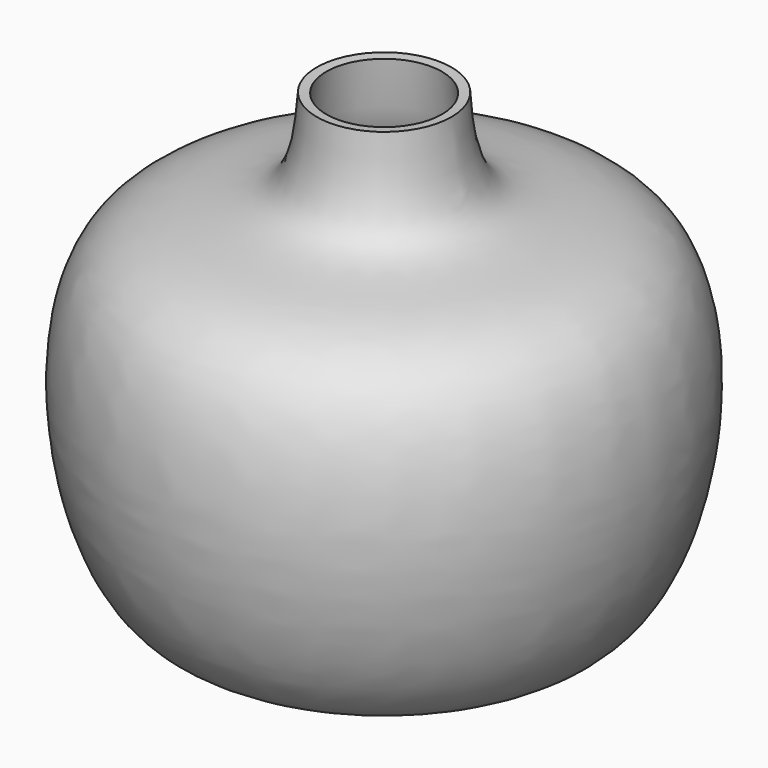
from build123d import *


# Not quite as in the source:
# - ends of sketch curves that miss each other by under 0.0002 mm in the source are joined
# - the dataset's text gives a spline's control points without its knots; the knots are read off the source's solid


with BuildPart() as f1:
    # F0 (on Front) → F1 (revolve)
    with BuildSketch(Plane.XZ):
        with BuildLine():
            add(Edge.make_bspline(
                [(0, 0), (12.2604930092, 0), (37.1680432505, -14.4897537862), (45.8159764504, 54.0703124701), (10.8709015607, 48.0211229848), (9.6057950827, 61.8857288852), (9.1015450487, 68.0656330135)],
                knots=[0, 0, 0, 0, 0.2642831779, 0.5818122538, 0.8089805027, 1, 1, 1, 1], degree=3))
            Line((0, 0), (0, -1.5000011719))
            add(Edge.make_bspline(
                [(0, -1.5000011719), (2.7725135208, -1.5000011719), (6.9145647776, -2.0308322394), (12.2903121109, -3.0792987233), (16.2230322301, -3.8437402004), (20.0419075684, -4.3880328646), (23.7428872911, -4.4983960181), (26.7225260222, -4.0210829824), (29.0016471213, -3.1616629238), (30.634715187, -2.2528712489), (32.1737960375, -1.0569174337), (33.5849093089, 0.4155370165), (34.8701777039, 2.1189441775), (36.4304008936, 4.6671279697), (38.1043575198, 8.3092557489), (39.6794960387, 13.2241653972), (40.8064070385, 18.4928093913), (41.4619597155, 23.9213048617), (41.6175636543, 29.3150527243), (41.2394176043, 34.481517293), (40.4444625408, 38.4415356728), (39.4887157156, 41.3119500081), (38.5996476038, 43.2930657424), (37.7032781151, 44.7799744639), (36.8819518489, 45.8554891408), (36.0025448677, 46.8394346131), (34.8057228996, 47.9062881725), (32.7340480289, 49.2933149411), (29.9423777814, 50.5045494733), (26.4845353427, 51.4020936649), (23.0859185409, 52.0045383585), (20.4473888451, 52.4533214053), (18.5513975566, 52.8808949316), (17.2640557934, 53.2558221623), (16.3263698889, 53.6258531422), (15.667143184, 53.9605779715), (15.0729428605, 54.3204393179), (14.4107406838, 54.8403517171), (13.7206126643, 55.5776441057), (13.1191641344, 56.4336487659), (12.4251973264, 57.7329037553), (11.7495447876, 59.6396265655), (11.2018431492, 62.2839868191), (10.8463357644, 65.168567942), (10.6789401827, 67.1782157689), (10.5965776894, 68.1876203849)],
                knots=[0, 0, 0, 0, 0.0625, 0.09375, 0.125, 0.15625, 0.1875, 0.21875, 0.234375, 0.25, 0.265625, 0.28125, 0.296875, 0.3125, 0.34375, 0.375, 0.40625, 0.4375, 0.46875, 0.5, 0.53125, 0.546875, 0.5625, 0.578125, 0.5859375, 0.59375, 0.609375, 0.625, 0.65625, 0.6875, 0.71875, 0.75, 0.765625, 0.78125, 0.796875, 0.8046875, 0.8125, 0.828125, 0.84375, 0.859375, 0.875, 0.90625, 0.9375, 0.96875, 0.9999999783, 0.9999999783, 0.9999999783, 0.9999999783], degree=3))
            Line((10.5965776894, 68.1876203849), (9.1015450487, 68.0656330135))
        make_face()
    revolve(axis=Axis((0, 0, 34.8241217434), (0, 0, -1)))


solid = f1.part
